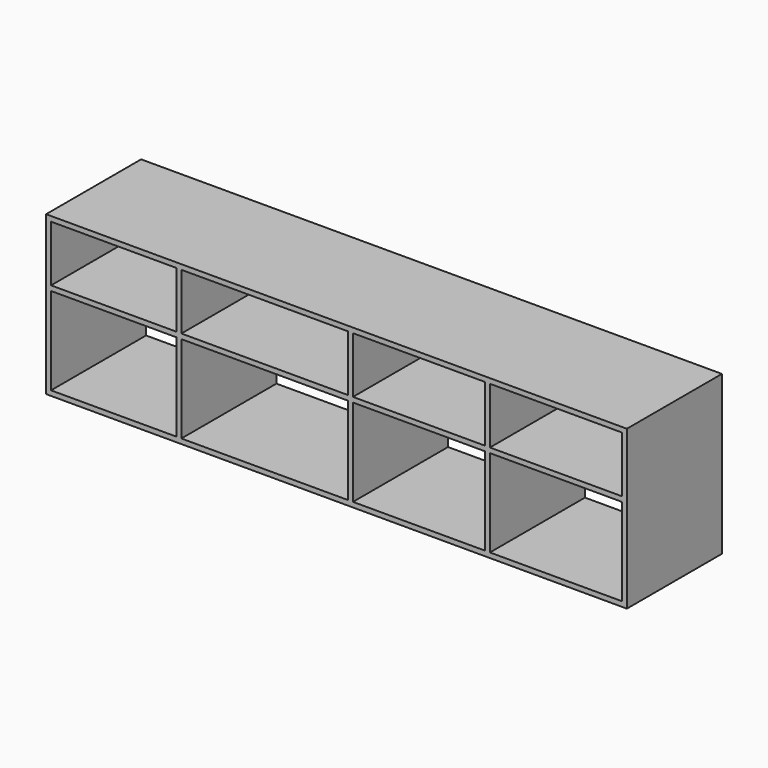
from build123d import *

# Parameters (mm, degrees)
F0_W     = 1117.6
F0_H     = 304.8
F0_W_2   = 9.525
F0_H_2   = 107.95
F1_DEPTH = 228.6
F0_W_3   = 320.675
F0_H_3   = 9.525
F0_W_4   = 254
F2_DEPTH = 228.6
F0_H_4   = 168.275
F3_DEPTH = 228.6
F4_DEPTH = 228.6
F5_DEPTH = 228.6


with BuildPart() as f1:
    # F0 (on Front) → F1 (new body)
    with BuildSketch(Plane.XZ):
        with Locations((43.0389853762, 152.4)):
            Rectangle(F0_W, F0_H)
        Polygon((-264.9360146238, 9.525), (-506.2360146238, 9.525), (-506.2360146238, 177.8), (-506.2360146238, 187.325), (-506.2360146238, 295.275), (-264.9360146238, 295.275), (-255.4110146238, 295.275), (65.2639853762, 295.275), (74.7889853762, 295.275), (328.7889853762, 295.275), (338.3139853762, 295.275), (592.3139853762, 295.275), (592.3139853762, 187.325), (592.3139853762, 177.8), (592.3139853762, 9.525), (338.3139853762, 9.525), (328.7889853762, 9.525), (74.7889853762, 9.525), (65.2639853762, 9.525), (-255.4110146238, 9.525), align=None, mode=Mode.SUBTRACT)
        Polygon((-506.2360146238, 187.325), (-506.2360146238, 177.8), (-264.9360146238, 177.8), (-264.9360146238, 9.525), (-255.4110146238, 9.525), (-255.4110146238, 177.8), (-255.4110146238, 187.325), (-264.9360146238, 187.325), align=None)
        with Locations((-260.1735146238, 241.3)):
            Rectangle(F0_W_2, F0_H_2)
    extrude(amount=F1_DEPTH)

    # F0 (on Front) → F2 (join, through all)
    with BuildSketch(Plane.XZ):
        with Locations((-95.0735146238, 182.5625)):
            Rectangle(F0_W_3, F0_H_3)
        with Locations((70.0264853762, 182.5625)):
            Rectangle(F0_W_2, F0_H_3)
        with Locations((201.7889853762, 182.5625)):
            Rectangle(F0_W_4, F0_H_3)
        with Locations((333.5514853762, 182.5625)):
            Rectangle(F0_W_2, F0_H_3)
        with Locations((465.3139853762, 182.5625)):
            Rectangle(F0_W_4, F0_H_3)
    extrude(amount=F2_DEPTH)

    # F0 (on Front) → F3 (join, through all)
    with BuildSketch(Plane.XZ):
        with Locations((333.5514853762, 93.6625)):
            Rectangle(F0_W_2, F0_H_4)
    extrude(amount=F3_DEPTH)

    # F0 (on Front) → F4 (join, through all)
    with BuildSketch(Plane.XZ):
        with Locations((-95.0735146238, 182.5625)):
            Rectangle(F0_W_3, F0_H_3)
        with Locations((70.0264853762, 93.6625)):
            Rectangle(F0_W_2, F0_H_4)
    extrude(amount=F4_DEPTH)

    # F0 (on Front) → F5 (join, through all)
    with BuildSketch(Plane.XZ):
        with Locations((70.0264853762, 241.3)):
            Rectangle(F0_W_2, F0_H_2)
        with Locations((333.5514853762, 241.3)):
            Rectangle(F0_W_2, F0_H_2)
    extrude(amount=F5_DEPTH)


solid = f1.part
